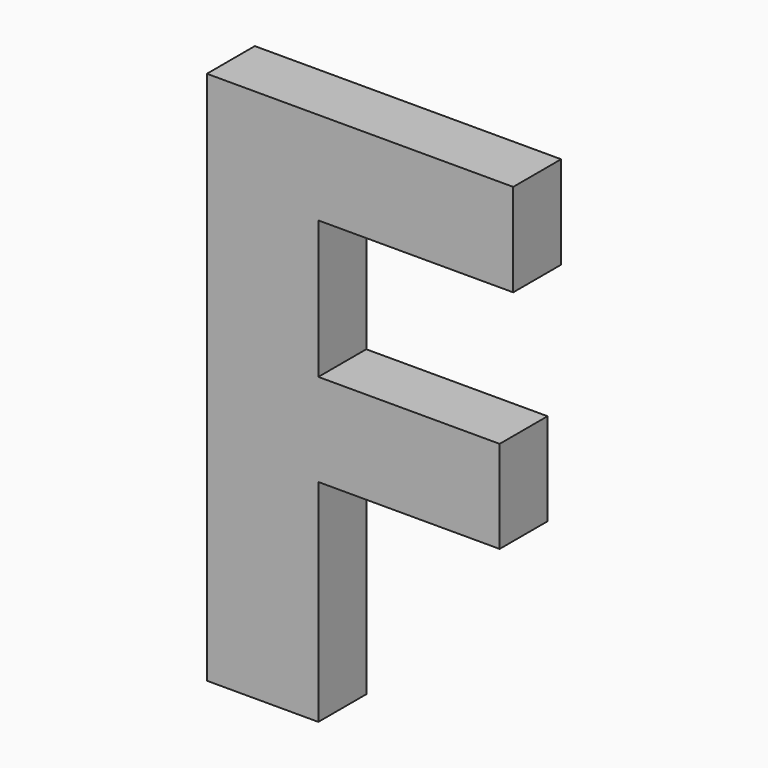
from build123d import *

# Parameters (mm, degrees)
F0_TEXT_SIZE = 62.5
F1_DEPTH     = 5


# Not quite as in the source:
# - Text() gives the source's letters only with a copy of the font that has no kerning and outlines rounded to 1/6400 em; it was checked with that copy


with BuildPart() as f1:
    # F0 (on Front) → F1 (new body)
    with BuildSketch(Plane.XZ):
        with Locations((-71.4473655724, 15.7894729022)):
            Text('F', F0_TEXT_SIZE, font='Open Sans', font_style=FontStyle.BOLD, text_align=(TextAlign.LEFT, TextAlign.BOTTOM))
    extrude(amount=F1_DEPTH)


solid = f1.part
